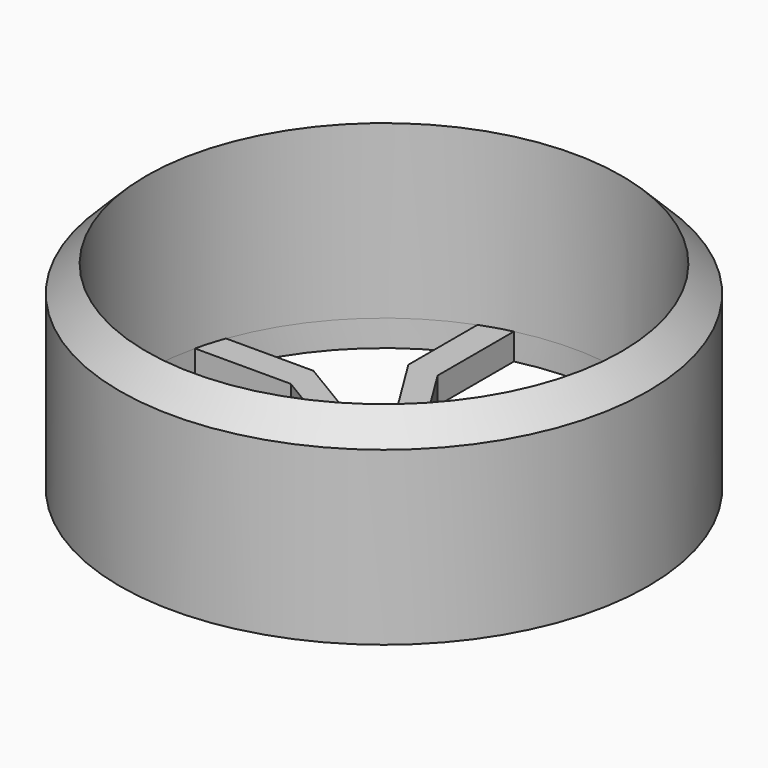
from build123d import *
from build123d import SkipClean  # not in build123d's __all__

# Parameters (mm, degrees)
F0_R     = 20
F1_DEPTH = 15
F2_R     = 18
F3_DEPTH = 13
F8_DEPTH = 25
F9_SIZE2 = 1.99999
F9_SIZE  = 1.99999


# Not quite as in the source:
# - a fillet or chamfer is up to 0.001 mm smaller than in the source, because OpenCascade refuses the exact size
# - the program builds the solid bodies; features that only make, move or delete a surface that nothing else refers to are left out


with BuildPart() as f1:
    # F0 (on Top) → F1 (new body)
    with BuildSketch(Plane.XY):
        Circle(F0_R)
    extrude(amount=F1_DEPTH)

    # F2 (on face) → F3 (cut)
    with BuildSketch(Plane.XY.offset(15)):
        Circle(F2_R)
    extrude(amount=-F3_DEPTH, mode=Mode.SUBTRACT)

    # F7 (on face) → F8 (cut)
    with BuildSketch(Plane(origin=(0, 0, 0), x_dir=(1, 0, 0), z_dir=(0, 0, -1))):
        with BuildLine():
            ThreePointArc((-4.17089, -17.510102), (-0.069604, -17.999865), (4.035348, -17.541835))
            Line((4.035348, -17.541835), (4.035348, -10.286759))
            Line((4.035348, -10.286759), (0, -3.568962))
            Line((0, -3.568962), (-4.17089, -10.286759))
            Line((-4.17089, -10.286759), (-4.17089, -17.510102))
        make_face()
        with BuildLine():
            Line((-6.386758, -10.286759), (-1.846161, -2.973498))
            ThreePointArc((-1.846161, -2.973498), (-2.49299, -2.456623), (-3.000305, -1.802269))
            Line((-3.000305, -1.802269), (-10.286759, -6.179206))
            Line((-10.286759, -6.179206), (-16.906135, -6.179206))
            ThreePointArc((-16.906135, -6.179206), (-12.805987, -12.649375), (-6.386758, -16.828824))
            Line((-6.386758, -16.828824), (-6.386758, -10.286759))
        make_face()
        with BuildLine():
            Line((-10.286759, 4.17089), (-17.510102, 4.17089))
            ThreePointArc((-17.510102, 4.17089), (-17.999865, 0.069604), (-17.541835, -4.035348))
            Line((-17.541835, -4.035348), (-10.286759, -4.035348))
            Line((-10.286759, -4.035348), (-3.568962, 0))
            Line((-3.568962, 0), (-10.286759, 4.17089))
        make_face()
        with BuildLine():
            ThreePointArc((-2.973498, 1.846161), (-2.456623, 2.49299), (-1.802269, 3.000305))
            Line((-1.802269, 3.000305), (-6.179206, 10.286759))
            Line((-6.179206, 10.286759), (-6.179206, 16.906135))
            ThreePointArc((-6.179206, 16.906135), (-12.649375, 12.805987), (-16.828824, 6.386758))
            Line((-16.828824, 6.386758), (-10.286759, 6.386758))
            Line((-10.286759, 6.386758), (-2.973498, 1.846161))
        make_face()
        with BuildLine():
            ThreePointArc((4.17089, 17.510102), (0.069604, 17.999865), (-4.035348, 17.541835))
            Line((-4.035348, 17.541835), (-4.035348, 10.286759))
            Line((-4.035348, 10.286759), (0, 3.568962))
            Line((0, 3.568962), (4.17089, 10.286759))
            Line((4.17089, 10.286759), (4.17089, 17.510102))
        make_face()
        with BuildLine():
            Line((6.386758, 10.286759), (1.846161, 2.973498))
            ThreePointArc((1.846161, 2.973498), (2.49299, 2.456623), (3.000305, 1.802269))
            Line((3.000305, 1.802269), (10.286759, 6.179206))
            Line((10.286759, 6.179206), (16.906135, 6.179206))
            ThreePointArc((16.906135, 6.179206), (12.805987, 12.649375), (6.386758, 16.828824))
            Line((6.386758, 16.828824), (6.386758, 10.286759))
        make_face()
        with BuildLine():
            ThreePointArc((18, 0), (17.885092, 2.030637), (17.541835, 4.035348))
            Line((17.541835, 4.035348), (10.286759, 4.035348))
            Line((10.286759, 4.035348), (3.568962, 0))
            Line((3.568962, 0), (10.286759, -4.17089))
            Line((10.286759, -4.17089), (17.510102, -4.17089))
            ThreePointArc((17.510102, -4.17089), (17.877106, -2.099781), (18, 0))
        make_face()
        with BuildLine():
            Line((10.286759, -6.386758), (2.973498, -1.846161))
            ThreePointArc((2.973498, -1.846161), (2.456623, -2.49299), (1.802269, -3.000305))
            Line((1.802269, -3.000305), (6.179206, -10.286759))
            Line((6.179206, -10.286759), (6.179206, -16.906135))
            ThreePointArc((6.179206, -16.906135), (12.649375, -12.805987), (16.828824, -6.386758))
            Line((16.828824, -6.386758), (10.286759, -6.386758))
        make_face()
    with SkipClean():  # cleaning this boolean's faces spoils the solid; the shape is the same uncleaned
        extrude(amount=-F8_DEPTH, mode=Mode.SUBTRACT)

    # F9 (size 2 and 2 in the source; OpenCascade refuses exactly that, so slightly less here)
    f9_edges = [f1.edges().sort_by_distance(p)[0] for p in [
        (-20, 0, 15),
    ]]
    chamfer(f9_edges, length=F9_SIZE, length2=F9_SIZE2)


solid = f1.part
